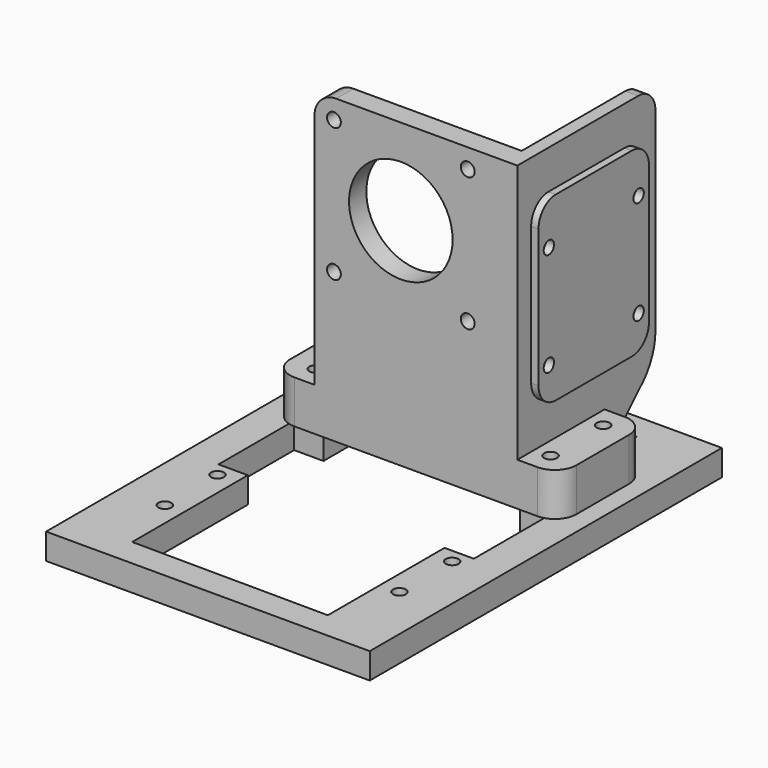
from build123d import *

# Parameters (mm, degrees)
F0_W         = 75
F0_H         = 102
F0_R         = 1.5
F1_DEPTH     = 6
F2_R         = 1.5
F3_DEPTH     = 10
F4_W         = 47
F4_H         = 5
F5_DEPTH     = 60
F6_R         = 12
F6_R_2       = 1.6
F7_DEPTH     = 25
F6_W         = 3
F6_H         = 60
F8_DEPTH     = 40
F9_R         = 1.5
F10_DEPTH    = 25
F11_T1_DEPTH = 3
F12_T1_DEPTH = 53.8871689707
F13_DEPTH    = 1.7
F14_R        = 5


# Not quite as in the source:
# - a fillet or chamfer that OpenCascade refuses, or shapes differently, is made with other operations: its cross-section is extruded or revolved along the edge and cut away or added


with BuildPart() as f1:
    # F0 (on Top) → F1 (new body)
    with BuildSketch(Plane.XY):
        Rectangle(F0_W, F0_H)
        with Locations((-27.185, -29.5)):
            Circle(F0_R, mode=Mode.SUBTRACT)
        with Locations((-27.185, -14.25)):
            Circle(F0_R, mode=Mode.SUBTRACT)
        with Locations((27.185, -29.5)):
            Circle(F0_R, mode=Mode.SUBTRACT)
        with Locations((27.185, -14.25)):
            Circle(F0_R, mode=Mode.SUBTRACT)
        with Locations((-27.185, 14.25)):
            Circle(F0_R, mode=Mode.SUBTRACT)
        with Locations((-27.185, 29.5)):
            Circle(F0_R, mode=Mode.SUBTRACT)
        Polygon((-22.785, 10.95), (-22.785, 44.45), (22.785, 44.75), (22.785, 10.95), (29.585, 10.95), (29.585, 0), (29.585, -10.95), (22.785, -10.95), (22.785, -44.75), (-22.785, -44.45), (-22.785, -10.95), (-29.585, -10.95), (-29.585, 0), (-29.585, 10.95), align=None, mode=Mode.SUBTRACT)
        with BuildLine():
            ThreePointArc((28.685, 14.25), (26.1243398282, 13.1893398282), (27.185, 15.75))
            ThreePointArc((27.185, 15.75), (28.2456601718, 15.3106601718), (28.685, 14.25))
        make_face(mode=Mode.SUBTRACT)
        with BuildLine():
            ThreePointArc((27.185, 28), (26.1243398282, 30.5606601718), (28.685, 29.5))
            ThreePointArc((28.685, 29.5), (28.2456601718, 28.4393398282), (27.185, 28))
        make_face(mode=Mode.SUBTRACT)
    extrude(amount=F1_DEPTH)


with BuildPart() as f3:
    # F2 (on face) → F3 (new body)
    with BuildSketch(Plane.XY.offset(6)):
        Polygon((-22.785, 34.5), (-33.185, 34.5), (-33.185, 9.25), (-29.585, 9.25), (-29.585, 10.95), (-22.785, 10.95), align=None)
        with Locations((-27.185, 14.25)):
            Circle(F2_R, mode=Mode.SUBTRACT)
        with Locations((-27.185, 29.5)):
            Circle(F2_R, mode=Mode.SUBTRACT)
        Polygon((22.785, 34.5), (-22.785, 34.5), (-22.785, 10.95), (-29.585, 10.95), (-29.585, 9.25), (29.585, 9.25), (29.585, 10.95), (22.785, 10.95), align=None)
        Polygon((33.185, 34.5), (22.785, 34.5), (22.785, 10.95), (29.585, 10.95), (29.585, 9.25), (33.185, 9.25), align=None)
        with Locations((27.185, 14.25)):
            Circle(F2_R, mode=Mode.SUBTRACT)
        with Locations((27.185, 29.5)):
            Circle(F2_R, mode=Mode.SUBTRACT)
    extrude(amount=F3_DEPTH)

    # F4 (on face) → F5 (join)
    with BuildSketch(Plane.XY.offset(16)):
        with Locations((0, 11.75)):
            Rectangle(F4_W, F4_H)
    extrude(amount=F5_DEPTH)

    # F6 (on face) → F7 (cut)
    with BuildSketch(Plane.XZ.offset(-9.25)):
        with Locations((-3.5, 56)):
            Circle(F6_R)
        with Locations((-19, 71.5)):
            Circle(F6_R_2)
        with Locations((12, 71.5)):
            Circle(F6_R_2)
        with Locations((12, 40.5)):
            Circle(F6_R_2)
        with Locations((-19, 40.5)):
            Circle(F6_R_2)
    extrude(amount=-F7_DEPTH, mode=Mode.SUBTRACT)

    # F6 (on face) → F8 (join)
    with BuildSketch(Plane.XZ.offset(-9.25)):
        with Locations((22, 46)):
            Rectangle(F6_W, F6_H)
    extrude(amount=-F8_DEPTH)

    # F9 (on face) → F10 (cut)
    with BuildSketch(Plane.YZ.offset(23.5)):
        with Locations((16.25, 57)):
            Circle(F9_R)
        with Locations((42.25, 57)):
            Circle(F9_R)
        with Locations((16.25, 33)):
            Circle(F9_R)
        with Locations((42.25, 33)):
            Circle(F9_R)
    extrude(amount=-F10_DEPTH, mode=Mode.SUBTRACT)

    # F11: chamfer of 10 on 2 edges, made by hand

    # F11_s2 → F11_t1 (join)
    with BuildSketch(Plane.YZ.offset(20.5)):
        Polygon((34.5, 6), (44.5, 16), (34.5, 16), align=None)
    extrude(amount=F11_T1_DEPTH)

    # F12: fillet of radius 13.2781745931 on 1 edges, made by hand

    # F12_s2 → F12_t1 (cut)
    with BuildSketch(Plane.YZ.offset(-4.9435844853)):
        with BuildLine():
            ThreePointArc((49.25, 26.1774337941), (48.0040428196, 20.5617713525), (44.5, 16))
            Line((44.5, 16), (49.25, 16))
            Line((49.25, 16), (49.25, 26.1774337941))
        make_face()
    extrude(amount=F12_T1_DEPTH, mode=Mode.SUBTRACT)

    # F14
    f14_edges = [f3.edges().sort_by_distance(p)[0] for p in [
        (22, 49.25, 76),
        (-23.5, 11.75, 76),
        (-33.185, 34.5, 11),
        (-33.185, 9.25, 11),
        (33.185, 9.25, 11),
        (33.185, 34.5, 11),
    ]]
    fillet(f14_edges, radius=F14_R)


with BuildPart() as f13:
    # F9 (on face) → F13 (new body)
    with BuildSketch(Plane.YZ.offset(23.5)):
        with BuildLine():
            Line((40.25, 67), (18.25, 67))
            ThreePointArc((18.25, 67), (14.7144660941, 65.5355339059), (13.25, 62))
            Line((13.25, 62), (13.25, 30))
            ThreePointArc((13.25, 30), (14.7144660941, 26.4644660941), (18.25, 25))
            Line((18.25, 25), (40.25, 25))
            ThreePointArc((40.25, 25), (43.7855339059, 26.4644660941), (45.25, 30))
            Line((45.25, 30), (45.25, 62))
            ThreePointArc((45.25, 62), (43.7855339059, 65.5355339059), (40.25, 67))
        make_face()
        with Locations((16.25, 33)):
            Circle(F9_R, mode=Mode.SUBTRACT)
        with Locations((42.25, 33)):
            Circle(F9_R, mode=Mode.SUBTRACT)
        with Locations((16.25, 57)):
            Circle(F9_R, mode=Mode.SUBTRACT)
        with Locations((42.25, 57)):
            Circle(F9_R, mode=Mode.SUBTRACT)
    extrude(amount=F13_DEPTH)


solid = Compound([f1.part, f3.part, f13.part])
